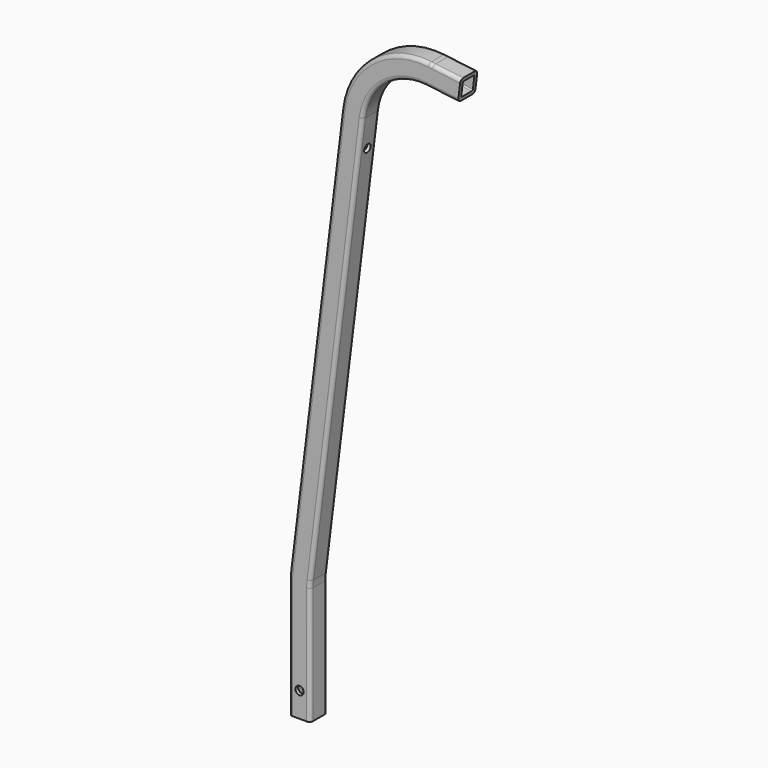
from build123d import *

# Parameters (mm, degrees)
F4_R      = 3.683
F5_DEPTH  = 334.01
F6_R      = 3.683
F7_DEPTH  = 25.4
F8_R      = 6.35
F9_DEPTH  = 9.4742
F11_DEPTH = 24.765
F12_R     = 6.35
F13_DEPTH = 12.446


# Not quite as in the source:
# - a feature names something its author has since deleted; it is built from what else it names


with BuildPart() as f2:
    # F2: sweep along a path in F0
    with BuildLine(Plane.XZ) as f2_path:
        Line((0, 0), (0, 104.902))
        ThreePointArc((0, 104.902), (0.1125182852, 108.5847531474), (0.4496534022, 112.2537681409))
        Line((0.4496534022, 112.2537681409), (46.8818732396, 490.4138519163))
        ThreePointArc((46.8818732396, 490.4138519163), (69.6174413383, 530.5988324867), (114.1089879783, 542.9374303731))
        Line((114.1089879783, 542.9374303731), (117.890588816, 542.4731081747))
    # F1 (on Top) → F2 (sweep)
    with BuildSketch(Plane.XY):
        with BuildLine():
            ThreePointArc((-9.525, -6.35), (-8.5950640303, -8.5950640303), (-6.35, -9.525))
            Line((-6.35, -9.525), (6.35, -9.525))
            ThreePointArc((6.35, -9.525), (8.5950640303, -8.5950640303), (9.525, -6.35))
            Line((9.525, -6.35), (9.525, 6.35))
            ThreePointArc((9.525, 6.35), (8.5950640303, 8.5950640303), (6.35, 9.525))
            Line((6.35, 9.525), (-6.35, 9.525))
            ThreePointArc((-6.35, 9.525), (-8.5950640303, 8.5950640303), (-9.525, 6.35))
            Line((-9.525, 6.35), (-9.525, -6.35))
        make_face()
        with BuildLine():
            Line((5.461, -6.477), (-5.461, -6.477))
            ThreePointArc((-5.461, -6.477), (-6.1794204897, -6.1794204897), (-6.477, -5.461))
            Line((-6.477, -5.461), (-6.477, 5.461))
            ThreePointArc((-6.477, 5.461), (-6.1794204897, 6.1794204897), (-5.461, 6.477))
            Line((-5.461, 6.477), (5.461, 6.477))
            ThreePointArc((5.461, 6.477), (6.1794204897, 6.1794204897), (6.477, 5.461))
            Line((6.477, 5.461), (6.477, -5.461))
            ThreePointArc((6.477, -5.461), (6.1794204897, -6.1794204897), (5.461, -6.477))
        make_face(mode=Mode.SUBTRACT)
    sweep(path=f2_path.line)

    # F4 (on Front) → F5 (cut, symmetric)
    with BuildSketch(Plane.XZ):
        with Locations((0, 22.225)):
            Circle(F4_R)
    extrude(amount=F5_DEPTH, both=True, mode=Mode.SUBTRACT)

    # F6 (on face) → F7 (cut)
    with BuildSketch(Plane(origin=(-22.5893491944, 0, 2.7736233219), x_dir=(0, -1, 0), z_dir=(-0.9925461516, 0, 0.1218693434))):
        with Locations((0, 464.5318445404)):
            Circle(F6_R)
    extrude(amount=-F7_DEPTH, mode=Mode.SUBTRACT)

    # F8 (on face) → F9 (cut)
    with BuildSketch(Plane(origin=(-22.5893491944, 0, 2.7736233219), x_dir=(0, -1, 0), z_dir=(-0.9925461516, 0, 0.1218693434))):
        with Locations((0, 464.5318445404)):
            Circle(F8_R)
    extrude(amount=-F9_DEPTH, mode=Mode.SUBTRACT)

    # F10 (on face) → F11 (join)
    with BuildSketch(Plane(origin=(50.5216003355, 0, -6.2032725133), x_dir=(0, 1, 0), z_dir=(0.9925461516, 0, -0.1218693434))):
        with BuildLine():
            ThreePointArc((9.525, 559.1468445404), (8.5950640303, 561.3919085707), (6.35, 562.3218445404))
            Line((6.35, 562.3218445404), (-6.35, 562.3218445404))
            ThreePointArc((-6.35, 562.3218445404), (-8.5950640303, 561.3919085707), (-9.525, 559.1468445404))
            Line((-9.525, 559.1468445404), (-9.525, 546.4468445404))
            ThreePointArc((-9.525, 546.4468445404), (-8.5950640303, 544.2017805101), (-6.35, 543.2718445404))
            Line((-6.35, 543.2718445404), (6.35, 543.2718445404))
            ThreePointArc((6.35, 543.2718445404), (8.5950640303, 544.2017805101), (9.525, 546.4468445404))
            Line((9.525, 546.4468445404), (9.525, 559.1468445404))
        make_face()
        with BuildLine():
            ThreePointArc((-6.477, 558.2578445404), (-6.1794204897, 558.9762650301), (-5.461, 559.2738445404))
            Line((-5.461, 559.2738445404), (5.461, 559.2738445404))
            ThreePointArc((5.461, 559.2738445404), (6.1794204897, 558.9762650301), (6.477, 558.2578445404))
            Line((6.477, 558.2578445404), (6.477, 547.3358445404))
            ThreePointArc((6.477, 547.3358445404), (6.1794204897, 546.6174240507), (5.461, 546.3198445404))
            Line((5.461, 546.3198445404), (-5.461, 546.3198445404))
            ThreePointArc((-5.461, 546.3198445404), (-6.1794204897, 546.6174240507), (-6.477, 547.3358445404))
            Line((-6.477, 547.3358445404), (-6.477, 558.2578445404))
        make_face(mode=Mode.SUBTRACT)
    extrude(amount=F11_DEPTH)

    # F12 (on face) → F13 (cut)
    with BuildSketch(Plane(origin=(0, 9.525, 0), x_dir=(-1, 0, 0), z_dir=(0, 1, 0))):
        with Locations((0, 22.225)):
            Circle(F12_R)
    extrude(amount=-F13_DEPTH, mode=Mode.SUBTRACT)


solid = f2.part
